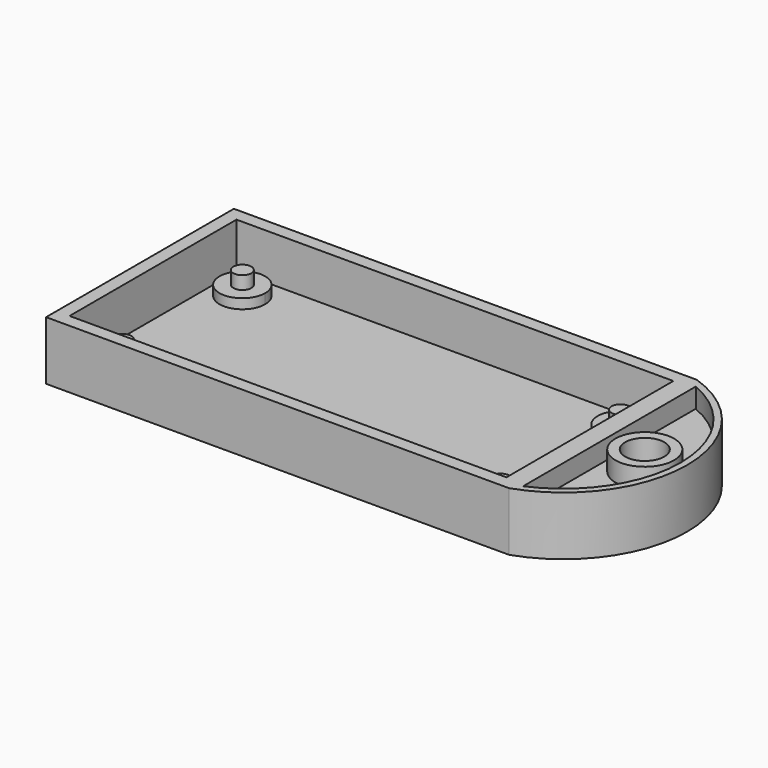
from build123d import *

# Parameters (mm, degrees)
F0_W     = 71
F0_H     = 36
F0_W_2   = 67
F0_H_2   = 32
F1_DEPTH = 7
F0_R     = 4.5
F0_R_2   = 3
F2_DEPTH = 2
F0_R_3   = 1.375
F3_DEPTH = 3.5
F4_DEPTH = 1.5
F5_DEPTH = 4


with BuildPart() as f1:
    # F0 (on Top) → F1 (new body)
    with BuildSketch(Plane.XY):
        Rectangle(F0_W, F0_H)
        Rectangle(F0_W_2, F0_H_2, mode=Mode.SUBTRACT)
        with BuildLine():
            ThreePointArc((35.5, -18), (48.4172374697, 0), (35.5, 18))
            Line((35.5, 18), (35.5, -18))
        make_face()
        with BuildLine():
            ThreePointArc((36.5, 16.5479447346), (47.4172374697, 0), (36.5, -16.5479447346))
            Line((36.5, -16.5479447346), (36.5, 16.5479447346))
        make_face(mode=Mode.SUBTRACT)
    extrude(amount=F1_DEPTH)

    # F0 (on Top) → F2 (join)
    with BuildSketch(Plane.XY):
        Rectangle(F0_W, F0_H)
        Rectangle(F0_W_2, F0_H_2, mode=Mode.SUBTRACT)
        Rectangle(F0_W_2, F0_H_2)
        Polygon((32.5, -11.5), (32.5, -15), (29, -15), (-29, -15), (-32.5, -15), (-32.5, -11.5), (-32.5, 11.5000000158), (-32.5, 15), (-29, 15), (29, 15), (32.5, 15), (32.5, 11.5), align=None, mode=Mode.SUBTRACT)
        with BuildLine():
            Line((-29, -15), (29, -15))
            ThreePointArc((29, -15), (26.5251262658, -9.0251262658), (32.5, -11.5))
            Line((32.5, -11.5), (32.5, 11.5))
            ThreePointArc((32.5, 11.5), (26.5251262658, 9.0251262658), (29, 15))
            Line((29, 15), (-29, 15))
            ThreePointArc((-29, 15), (-26.5251262658, 13.9748737342), (-25.5, 11.5))
            ThreePointArc((-25.5, 11.5), (-29.0000000079, 8), (-32.5, 11.5000000158))
            Line((-32.5, 11.5000000158), (-32.5, -11.5))
            ThreePointArc((-32.5, -11.5), (-29, -8), (-25.5, -11.5))
            ThreePointArc((-25.5, -11.5), (-26.5251262658, -13.9748737342), (-29, -15))
        make_face()
        with BuildLine():
            ThreePointArc((35.5, -18), (48.4172374697, 0), (35.5, 18))
            Line((35.5, 18), (35.5, -18))
        make_face()
        with BuildLine():
            ThreePointArc((36.5, 16.5479447346), (47.4172374697, 0), (36.5, -16.5479447346))
            Line((36.5, -16.5479447346), (36.5, 16.5479447346))
        make_face(mode=Mode.SUBTRACT)
        with BuildLine():
            Line((36.5, 16.5479447346), (36.5, -16.5479447346))
            ThreePointArc((36.5, -16.5479447346), (47.4172374697, 0), (36.5, 16.5479447346))
        make_face()
        with Locations((41.9172374697, 0)):
            Circle(F0_R, mode=Mode.SUBTRACT)
        with Locations((41.9172374697, 0)):
            Circle(F0_R)
        with Locations((41.9172374697, 0)):
            Circle(F0_R_2, mode=Mode.SUBTRACT)
        with BuildLine():
            Line((29, -15), (32.5, -15))
            Line((32.5, -15), (32.5, -11.5))
            ThreePointArc((32.5, -11.5), (31.4748737342, -13.9748737342), (29, -15))
        make_face()
        with BuildLine():
            Line((-32.5, -15), (-29, -15))
            ThreePointArc((-29, -15), (-31.4748737342, -13.9748737342), (-32.5, -11.5))
            Line((-32.5, -11.5), (-32.5, -15))
        make_face()
        with BuildLine():
            Line((-32.5, 15), (-32.5, 11.5000000158))
            ThreePointArc((-32.5, 11.5000000158), (-31.4748737286, 13.9748737397), (-29, 15))
            Line((-29, 15), (-32.5, 15))
        make_face()
        with BuildLine():
            ThreePointArc((29, 15), (31.4748737342, 13.9748737342), (32.5, 11.5))
            Line((32.5, 11.5), (32.5, 15))
            Line((32.5, 15), (29, 15))
        make_face()
    extrude(amount=-F2_DEPTH)


with BuildPart() as f1b:
    # F0 (on Top) → F1, piece 2 (new body)
    with BuildSketch(Plane.XY):
        with Locations((41.9172374697, 0)):
            Circle(F0_R)
        with Locations((41.9172374697, 0)):
            Circle(F0_R_2, mode=Mode.SUBTRACT)
    extrude(amount=F1_DEPTH)


with BuildPart() as f2:
    # F0 (on Top) → F2, piece 2 (new body)
    with BuildSketch(Plane.XY):
        with Locations((29, -11.5)):
            Circle(F0_R_3)
    extrude(amount=-F2_DEPTH)


with BuildPart() as f2b:
    # F0 (on Top) → F2, piece 3 (new body)
    with BuildSketch(Plane.XY):
        with Locations((29, 11.5)):
            Circle(F0_R_3)
    extrude(amount=-F2_DEPTH)


with BuildPart() as f2c:
    # F0 (on Top) → F2, piece 4 (new body)
    with BuildSketch(Plane.XY):
        with Locations((-29, -11.5)):
            Circle(F0_R_3)
    extrude(amount=-F2_DEPTH)


with BuildPart() as f2d:
    # F0 (on Top) → F2, piece 5 (new body)
    with BuildSketch(Plane.XY):
        with Locations((-29, 11.5)):
            Circle(F0_R_3)
    extrude(amount=-F2_DEPTH)


with BuildPart() as f3:
    # F0 (on Top) → F3 (new body)
    with BuildSketch(Plane.XY):
        with Locations((29, 11.5)):
            Circle(F0_R_3)
    extrude(amount=F3_DEPTH)


with BuildPart() as f3b:
    # F0 (on Top) → F3, piece 2 (new body)
    with BuildSketch(Plane.XY):
        with Locations((29, -11.5)):
            Circle(F0_R_3)
    extrude(amount=F3_DEPTH)


with BuildPart() as f3c:
    # F0 (on Top) → F3, piece 3 (new body)
    with BuildSketch(Plane.XY):
        with Locations((-29, -11.5)):
            Circle(F0_R_3)
    extrude(amount=F3_DEPTH)


with BuildPart() as f3d:
    # F0 (on Top) → F3, piece 4 (new body)
    with BuildSketch(Plane.XY):
        with Locations((-29, 11.5)):
            Circle(F0_R_3)
    extrude(amount=F3_DEPTH)


with BuildPart() as f4:
    # F0 (on Top) → F4 (new body)
    with BuildSketch(Plane.XY):
        with BuildLine():
            ThreePointArc((-29, 15), (-31.4748737286, 13.9748737397), (-32.5, 11.5000000158))
            ThreePointArc((-32.5, 11.5000000158), (-29.0000000079, 8), (-25.5, 11.5))
            ThreePointArc((-25.5, 11.5), (-26.5251262658, 13.9748737342), (-29, 15))
        make_face()
        with Locations((-29, 11.5)):
            Circle(F0_R_3, mode=Mode.SUBTRACT)
    extrude(amount=F4_DEPTH)


with BuildPart() as f4b:
    # F0 (on Top) → F4, piece 2 (new body)
    with BuildSketch(Plane.XY):
        with BuildLine():
            ThreePointArc((29, 15), (26.5251262658, 9.0251262658), (32.5, 11.5))
            ThreePointArc((32.5, 11.5), (31.4748737342, 13.9748737342), (29, 15))
        make_face()
        with Locations((29, 11.5)):
            Circle(F0_R_3, mode=Mode.SUBTRACT)
    extrude(amount=F4_DEPTH)


with BuildPart() as f4c:
    # F0 (on Top) → F4, piece 3 (new body)
    with BuildSketch(Plane.XY):
        with BuildLine():
            ThreePointArc((32.5, -11.5), (26.5251262658, -9.0251262658), (29, -15))
            ThreePointArc((29, -15), (31.4748737342, -13.9748737342), (32.5, -11.5))
        make_face()
        with Locations((29, -11.5)):
            Circle(F0_R_3, mode=Mode.SUBTRACT)
    extrude(amount=F4_DEPTH)


with BuildPart() as f4d:
    # F0 (on Top) → F4, piece 4 (new body)
    with BuildSketch(Plane.XY):
        with BuildLine():
            ThreePointArc((-32.5, -11.5), (-31.4748737342, -13.9748737342), (-29, -15))
            ThreePointArc((-29, -15), (-26.5251262658, -13.9748737342), (-25.5, -11.5))
            ThreePointArc((-25.5, -11.5), (-29, -8), (-32.5, -11.5))
        make_face()
        with Locations((-29, -11.5)):
            Circle(F0_R_3, mode=Mode.SUBTRACT)
    extrude(amount=F4_DEPTH)


with BuildPart() as f5:
    # F0 (on Top) → F5 (new body)
    with BuildSketch(Plane.XY):
        with BuildLine():
            Line((36.5, 16.5479447346), (36.5, -16.5479447346))
            ThreePointArc((36.5, -16.5479447346), (47.4172374697, 0), (36.5, 16.5479447346))
        make_face()
        with Locations((41.9172374697, 0)):
            Circle(F0_R, mode=Mode.SUBTRACT)
    extrude(amount=F5_DEPTH)


solid = Compound([f1.part, f1b.part, f2.part, f2b.part, f2c.part, f2d.part, f3.part, f3b.part, f3c.part, f3d.part, f4.part, f4b.part, f4c.part, f4d.part, f5.part])
